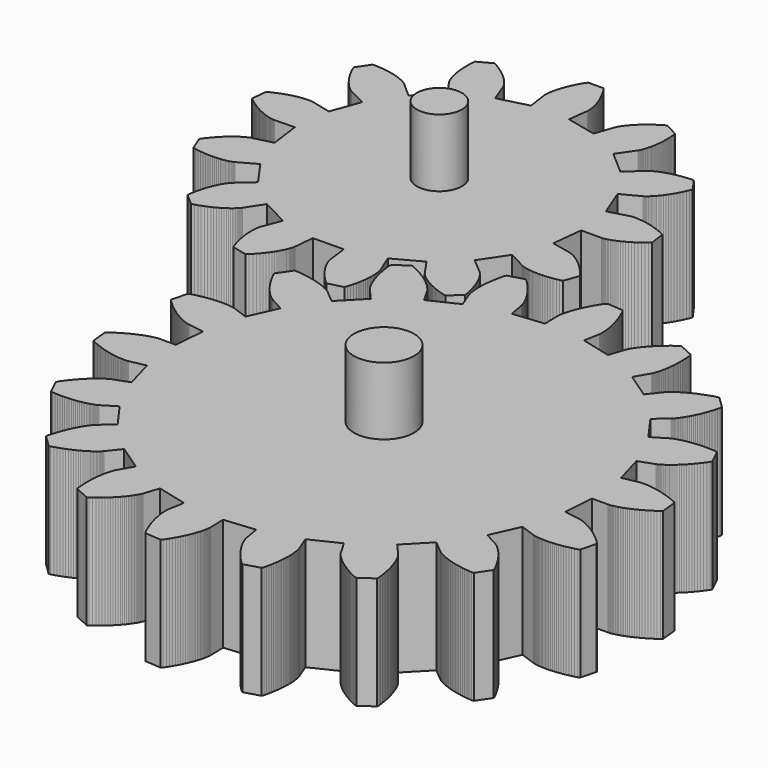
from build123d import *

# Parameters (mm, degrees)
F1_DEPTH = 25
F2_SCALE = 0.3
F3_R     = 1.5
F4_DEPTH = 12
F3_R_2   = 2


# Not quite as in the source:
# - the program builds the solid bodies; features that only make, move or delete a surface that nothing else refers to are left out


with BuildPart() as f1:
    # F0 (on Top) → F1 (new body)
    with BuildSketch(Plane.XY):
        Polygon((63.128658, -38.192269), (63.636659, -31.363161), (67.214568, -31.36309), (67.240708, -31.362349), (67.285548, -31.360198), (67.348975, -31.355999), (67.430963, -31.348944), (67.531399, -31.338361), (67.650141, -31.323509), (67.787089, -31.303718), (67.942102, -31.278212), (68.11496, -31.246286), (68.305495, -31.207304), (68.513461, -31.160525), (68.738673, -31.10528), (68.98082, -31.040863), (69.239687, -30.966603), (69.514891, -30.881866), (69.806179, -30.785946), (70.113202, -30.678172), (70.435603, -30.557981), (70.773002, -30.424666), (71.125005, -30.277628), (71.491224, -30.116233), (71.871164, -29.939914), (72.264438, -29.748074), (72.670593, -29.540111), (73.089091, -29.315462), (73.519448, -29.073598), (73.961158, -28.813953), (74.413704, -28.536), (74.876514, -28.239208), (75.349025, -27.923119), (75.830634, -27.587239), (76.133425, -27.244269), (75.778317, -23.714939), (75.413266, -23.439137), (74.874361, -23.205951), (74.348371, -22.990333), (73.835713, -22.791719), (73.336885, -22.609474), (72.852311, -22.443034), (72.382373, -22.291763), (71.927502, -22.154991), (71.48808, -22.032083), (71.064468, -21.922439), (70.65701, -21.825355), (70.265992, -21.740159), (69.891763, -21.666217), (69.534539, -21.602787), (69.194675, -21.549201), (68.872343, -21.504786), (68.567786, -21.468802), (68.281191, -21.44058), (68.012727, -21.419379), (67.762608, -21.404491), (67.530903, -21.395213), (67.317792, -21.390803), (67.123306, -21.390556), (66.947552, -21.393731), (66.790563, -21.399623), (66.652415, -21.40749), (66.533069, -21.416592), (66.432564, -21.426222), (66.350824, -21.435641), (66.287821, -21.444144), (66.243477, -21.451022), (66.217687, -21.455503), (62.7115, -22.168184), (60.853173, -15.577202), (64.215252, -14.353416), (64.239594, -14.34375), (64.28101, -14.326429), (64.339184, -14.300782), (64.413792, -14.266103), (64.504527, -14.22183), (64.611067, -14.167255), (64.732985, -14.101779), (64.869901, -14.024803), (65.021421, -13.935727), (65.187119, -13.833915), (65.366576, -13.718804), (65.559297, -13.589863), (65.764829, -13.44653), (65.982667, -13.288204), (66.212288, -13.114425), (66.453202, -12.924665), (66.704872, -12.718397), (66.966704, -12.495194), (67.238135, -12.254493), (67.518625, -11.995943), (67.80755, -11.719047), (68.104307, -11.423421), (68.408262, -11.108637), (68.71874, -10.774309), (69.035183, -10.420085), (69.356879, -10.045576), (69.68313, -9.650535), (70.013332, -9.23454), (70.346704, -8.797413), (70.682622, -8.338767), (71.020301, -7.858424), (71.187549, -7.432551), (69.646757, -4.237548), (69.209386, -4.10321), (68.623246, -4.068391), (68.055204, -4.045672), (67.505539, -4.034384), (66.974467, -4.033749), (66.462165, -4.043096), (65.968838, -4.061654), (65.494637, -4.088711), (65.03969, -4.123531), (64.604117, -4.16537), (64.188014, -4.213488), (63.791457, -4.267181), (63.414483, -4.325672), (63.057119, -4.388219), (62.719402, -4.454118), (62.401337, -4.522629), (62.102816, -4.593006), (61.823877, -4.664481), (61.564372, -4.736376), (61.324236, -4.807956), (61.103327, -4.878475), (60.901538, -4.947232), (60.718693, -5.013518), (60.554652, -5.076595), (60.409132, -5.135827), (60.282024, -5.190472), (60.172982, -5.239825), (60.081824, -5.283287), (60.008233, -5.320083), (59.95193, -5.349646), (59.912597, -5.371234), (59.889913, -5.384288), (56.83895, -7.253163), (52.838414, -1.695255), (55.579181, 0.604645), (55.598759, 0.622037), (55.631743, 0.65248), (55.677641, 0.696472), (55.735884, 0.754573), (55.806016, 0.827246), (55.887436, 0.914948), (55.979619, 1.018169), (56.08196, 1.13734), (56.193896, 1.272875), (56.314792, 1.425204), (56.444051, 1.594714), (56.581033, 1.781828), (56.725143, 1.986828), (56.875673, 2.210064), (57.032026, 2.451929), (57.193526, 2.712631), (57.359437, 2.992526), (57.529159, 3.291859), (57.701914, 3.61084), (57.877068, 3.949754), (58.053847, 4.308776), (58.231576, 4.688046), (58.409515, 5.087815), (58.586965, 5.508184), (58.763176, 5.949263), (58.937377, 6.411189), (59.108862, 6.894038), (59.276856, 7.39784), (59.440616, 7.922665), (59.5994, 8.468519), (59.752435, 9.035399), (59.763936, 9.492776), (57.223302, 11.968147), (56.766382, 11.944758), (56.203666, 11.777011), (55.662119, 11.604078), (55.141734, 11.426701), (54.642484, 11.245656), (54.164259, 11.061648), (53.707024, 10.875486), (53.270674, 10.687879), (52.855066, 10.499567), (52.460096, 10.311255), (52.085515, 10.123718), (51.731257, 9.937626), (51.396999, 9.75376), (51.082605, 9.57275), (50.787823, 9.395301), (50.512339, 9.222158), (50.255905, 9.053919), (50.018202, 8.891359), (49.798951, 8.735043), (49.597763, 8.585642), (49.414317, 8.443825), (49.248231, 8.310193), (49.099075, 8.185381), (48.9665, 8.069986), (48.850016, 7.964577), (48.749225, 7.869751), (48.663677, 7.78607), (48.592874, 7.71407), (48.536324, 7.654308), (48.493532, 7.607283), (48.463934, 7.573521), (48.447072, 7.553521), (46.219279, 4.753804), (40.559138, 8.608325), (42.348004, 11.706914), (42.360419, 11.729951), (42.381023, 11.769814), (42.409068, 11.826857), (42.443958, 11.901401), (42.485022, 11.993651), (42.531552, 12.103929), (42.582846, 12.232447), (42.638269, 12.379413), (42.697075, 12.545079), (42.758565, 12.729545), (42.822065, 12.933064), (42.8868, 13.155736), (42.952098, 13.397635), (43.017222, 13.658938), (43.081427, 13.939678), (43.143974, 14.239891), (43.204193, 14.55965), (43.261274, 14.898986), (43.314509, 15.257836), (43.36319, 15.636188), (43.406512, 16.034016), (43.4438, 16.451212), (43.474316, 16.887738), (43.497282, 17.343454), (43.511994, 17.818188), (43.517673, 18.311832), (43.513687, 18.824204), (43.499223, 19.355099), (43.473646, 19.904269), (43.436145, 20.471504), (43.386086, 21.056545), (43.240423, 21.490288), (40.006405, 22.947402), (39.585012, 22.769145), (39.11363, 22.419048), (38.663909, 22.071347), (38.235566, 21.726686), (37.82832, 21.385794), (37.441886, 21.049354), (37.075915, 20.718022), (36.730016, 20.392476), (36.403909, 20.07339), (36.097134, 19.761324), (35.809301, 19.45702), (35.540027, 19.160968), (35.288848, 18.873841), (35.05531, 18.596241), (34.838986, 18.32866), (34.63935, 18.071731), (34.455905, 17.82595), (34.28816, 17.591883), (34.135582, 17.370019), (33.997612, 17.160821), (33.873751, 16.964822), (33.763367, 16.782431), (33.665895, 16.614122), (33.580805, 16.460347), (33.507392, 16.321461), (33.445126, 16.197879), (33.393338, 16.089967), (33.351429, 15.998101), (33.318726, 15.92261), (33.294596, 15.863801), (33.278369, 15.82196), (33.269337, 15.79737), (32.133464, 12.404568), (25.496337, 14.09074), (26.117544, 17.614281), (26.121354, 17.640179), (26.127033, 17.684696), (26.133913, 17.747913), (26.141215, 17.829864), (26.148235, 17.930584), (26.154233, 18.050107), (26.158501, 18.188428), (26.160265, 18.345519), (26.158889, 18.521273), (26.153563, 18.715689), (26.143614, 18.928628), (26.128339, 19.160015), (26.106925, 19.409677), (26.078774, 19.677468), (26.043073, 19.963217), (25.999187, 20.266746), (25.946376, 20.587813), (25.88397, 20.926197), (25.811297, 21.281618), (25.727618, 21.653801), (25.632262, 22.042456), (25.524595, 22.447266), (25.40398, 22.867885), (25.269678, 23.303953), (25.121123, 23.755121), (24.957681, 24.220962), (24.778681, 24.701058), (24.583525, 25.194982), (24.371611, 25.702278), (24.142376, 26.222482), (23.895255, 26.75511), (23.610034, 27.112862), (20.072697, 27.375997), (19.737699, 27.064388), (19.414448, 26.574205), (19.110777, 26.093614), (18.826156, 25.623256), (18.560056, 25.163659), (18.311983, 24.715312), (18.081407, 24.278786), (17.86773, 23.854603), (17.670421, 23.443194), (17.488846, 23.045049), (17.322476, 22.66063), (17.170711, 22.290353), (17.032881, 21.934646), (16.908386, 21.5939), (16.79659, 21.268462), (16.69686, 20.958759), (16.60856, 20.665069), (16.530984, 20.387718), (16.463498, 20.127048), (16.405395, 19.88328), (16.356041, 19.656728), (16.314696, 19.4476), (16.280688, 19.256112), (16.253277, 19.082473), (16.231828, 18.926863), (16.215565, 18.789457), (16.203818, 18.670359), (16.195845, 18.569676), (16.190941, 18.487548), (16.188401, 18.424013), (16.187449, 18.379141), (16.187378, 18.352964), (16.280406, 14.776292), (9.466821, 14.09074), (8.845438, 17.614249), (8.840181, 17.639893), (8.830304, 17.683673), (8.815134, 17.74541), (8.793967, 17.824927), (8.766098, 17.921977), (8.730855, 18.036349), (8.68757, 18.16779), (8.635535, 18.315993), (8.574116, 18.480707), (8.502608, 18.661574), (8.420446, 18.858246), (8.326925, 19.070442), (8.221444, 19.297738), (8.10337, 19.539745), (7.972101, 19.796071), (7.827039, 20.066301), (7.667619, 20.349935), (7.493241, 20.646547), (7.303375, 20.95569), (7.097424, 21.276789), (6.874927, 21.609419), (6.63532, 21.952992), (6.378075, 22.30697), (6.102766, 22.670826), (5.808867, 23.043956), (5.495918, 23.425802), (5.163496, 23.815695), (4.811212, 24.213098), (4.438573, 24.617348), (4.045226, 25.027766), (3.630818, 25.443761), (3.240469, 25.682383), (-0.173573, 24.719828), (-0.381782, 24.312403), (-0.517849, 23.741222), (-0.638852, 23.185776), (-0.74546, 22.646414), (-0.838277, 22.123524), (-0.918039, 21.617396), (-0.985456, 21.128338), (-1.04116, 20.65664), (-1.085856, 20.202544), (-1.120287, 19.766336), (-1.145122, 19.348187), (-1.161139, 18.948314), (-1.169007, 18.566926), (-1.169429, 18.20413), (-1.163185, 17.860132), (-1.150944, 17.53498), (-1.133482, 17.228802), (-1.111538, 16.941643), (-1.085786, 16.673603), (-1.056999, 16.424679), (-1.025919, 16.19488), (-0.993252, 15.98424), (-0.959704, 15.792644), (-0.926048, 15.620136), (-0.892993, 15.466571), (-0.861277, 15.331884), (-0.831574, 15.215924), (-0.804657, 15.118627), (-0.781162, 15.039745), (-0.76183, 14.979176), (-0.747401, 14.936699), (-0.738511, 14.912078), (0.5722, 11.582912), (-5.59598, 8.608325), (-7.384986, 11.706807), (-7.39871, 11.729103), (-7.422944, 11.766886), (-7.458329, 11.819695), (-7.505424, 11.887184), (-7.564795, 11.968852), (-7.637046, 12.064278), (-7.722664, 12.172968), (-7.822254, 12.294464), (-7.936306, 12.428204), (-8.065352, 12.573724), (-8.209852, 12.730463), (-8.370294, 12.897857), (-8.547178, 13.075373), (-8.740886, 13.26238), (-8.95192, 13.45835), (-9.180626, 13.662679), (-9.427464, 13.874662), (-9.692753, 14.093771), (-9.976914, 14.319306), (-10.280233, 14.550623), (-10.603095, 14.787085), (-10.945783, 15.028), (-11.308581, 15.27265), (-11.691732, 15.520406), (-12.095521, 15.770488), (-12.520197, 16.02227), (-12.965895, 16.274995), (-13.432902, 16.527903), (-13.921287, 16.780315), (-14.431299, 17.031495), (-14.962971, 17.280662), (-15.41142, 17.371359), (-18.290336, 15.299177), (-18.346639, 14.845157), (-18.279188, 14.261837), (-18.202917, 13.698521), (-18.118603, 13.155243), (-18.026985, 12.632108), (-17.928843, 12.129224), (-17.824879, 11.646625), (-17.715907, 11.184309), (-17.602595, 10.742314), (-17.485755, 10.320637), (-17.366127, 9.919211), (-17.244383, 9.537966), (-17.121299, 9.176898), (-16.99765, 8.835831), (-16.874108, 8.514697), (-16.751412, 8.213356), (-16.630303, 7.931593), (-16.511453, 7.669303), (-16.395566, 7.426203), (-16.283382, 7.202153), (-16.175572, 6.996871), (-16.072844, 6.810077), (-15.975794, 6.641518), (-15.885167, 6.490919), (-15.801593, 6.357922), (-15.72571, 6.24221), (-15.658154, 6.143397), (-15.599557, 6.061164), (-15.550521, 5.995089), (-15.511646, 5.944782), (-15.483528, 5.909787), (-15.466736, 5.889714), (-13.096459, 3.209627), (-17.875256, -1.695255), (-20.616163, 0.604502), (-20.636658, 0.620766), (-20.672361, 0.647964), (-20.72369, 0.685502), (-20.790999, 0.732807), (-20.87475, 0.789253), (-20.975255, 0.854199), (-21.092908, 0.927049), (-21.22802, 1.007164), (-21.38095, 1.09384), (-21.551977, 1.186446), (-21.741382, 1.284305), (-21.94938, 1.386716), (-22.176288, 1.493043), (-22.422316, 1.602546), (-22.68764, 1.714517), (-22.972436, 1.828254), (-23.276883, 1.943083), (-23.601123, 2.05823), (-23.945291, 2.172954), (-24.309464, 2.286583), (-24.693711, 2.398342), (-25.0981, 2.507527), (-25.522703, 2.613361), (-25.967484, 2.715102), (-26.43248, 2.812046), (-26.917622, 2.903379), (-27.422904, 2.988398), (-27.948228, 3.066362), (-28.493516, 3.136494), (-29.058663, 3.198091), (-29.6435, 3.250373), (-30.095938, 3.182252), (-32.092484, 0.250384), (-31.990105, -0.195527), (-31.727218, -0.720565), (-31.462844, -1.223837), (-31.197841, -1.705521), (-30.932832, -2.165756), (-30.668599, -2.604753), (-30.405851, -3.022723), (-30.145327, -3.419881), (-29.887693, -3.79647), (-29.633655, -4.152742), (-29.383928, -4.489045), (-29.13917, -4.805628), (-28.900021, -5.102842), (-28.667155, -5.381042), (-28.441232, -5.640547), (-28.222861, -5.881776), (-28.012678, -6.105118), (-27.811312, -6.310965), (-27.619296, -6.499737), (-27.437229, -6.671927), (-27.265706, -6.827961), (-27.105264, -6.968329), (-26.956463, -7.093532), (-26.81976, -7.204057), (-26.695758, -7.300472), (-26.584845, -7.383232), (-26.487585, -7.452976), (-26.4044, -7.510197), (-26.335713, -7.55553), (-26.281986, -7.589502), (-26.243603, -7.612786), (-26.220956, -7.625909), (-23.076965, -9.33367), (-25.890015, -15.577202), (-29.252164, -14.353556), (-29.277001, -14.345302), (-29.31986, -14.331967), (-29.380924, -14.314222), (-29.460372, -14.292808), (-29.558342, -14.268432), (-29.675001, -14.241762), (-29.810469, -14.21354), (-29.964847, -14.184471), (-30.1382, -14.155331), (-30.33057, -14.126791), (-30.542024, -14.099627), (-30.772528, -14.07451), (-31.02212, -14.052214), (-31.290762, -14.033481), (-31.578379, -14.018982), (-31.884906, -14.009492), (-32.210241, -14.005754), (-32.554342, -14.008469), (-32.91696, -14.018347), (-33.29803, -14.036127), (-33.697338, -14.062516), (-34.114712, -14.098252), (-34.549865, -14.144007), (-35.002653, -14.200521), (-35.472731, -14.268467), (-35.959878, -14.348582), (-36.46375, -14.44147), (-36.984062, -14.547903), (-37.520463, -14.668481), (-38.072561, -14.803912), (-38.640038, -14.954795), (-39.041887, -15.173554), (-39.915262, -18.611479), (-39.666553, -18.995478), (-39.239937, -19.39895), (-38.819393, -19.781466), (-38.405616, -20.143452), (-37.999181, -20.485293), (-37.600755, -20.80745), (-37.2109, -21.11031), (-36.830254, -21.394402), (-36.459341, -21.660185), (-36.098769, -21.908116), (-35.749097, -22.138692), (-35.410784, -22.352475), (-35.084425, -22.549996), (-34.770453, -22.731747), (-34.469395, -22.898364), (-34.181703, -23.050341), (-33.907807, -23.188312), (-33.64816, -23.312843), (-33.40316, -23.424602), (-33.173183, -23.524121), (-32.958656, -23.612104), (-32.759869, -23.689115), (-32.577198, -23.755861), (-32.410972, -23.813011), (-32.261466, -23.861165), (-32.128926, -23.901029), (-32.013672, -23.933273), (-31.915917, -23.958602), (-31.83591, -23.977688), (-31.773786, -23.99127), (-31.729758, -23.999983), (-31.704006, -24.004604), (-28.1655, -24.534053), (-28.673501, -31.363161), (-32.25141, -31.363231), (-32.27755, -31.363972), (-32.32239, -31.366124), (-32.385818, -31.370322), (-32.467805, -31.377378), (-32.568241, -31.387961), (-32.686983, -31.402813), (-32.823931, -31.422604), (-32.978945, -31.44811), (-33.151802, -31.480036), (-33.342338, -31.519018), (-33.550303, -31.565796), (-33.775515, -31.621041), (-34.017662, -31.685459), (-34.276529, -31.759718), (-34.551733, -31.844456), (-34.843021, -31.940376), (-35.150044, -32.048149), (-35.472445, -32.168341), (-35.809844, -32.301656), (-36.161847, -32.448693), (-36.528066, -32.610089), (-36.908006, -32.786408), (-37.30128, -32.978248), (-37.707435, -33.186211), (-38.125933, -33.41086), (-38.55629, -33.652724), (-38.998, -33.912368), (-39.450546, -34.190322), (-39.913357, -34.487114), (-40.385868, -34.803203), (-40.867476, -35.139082), (-41.170267, -35.482053), (-40.815159, -39.011383), (-40.450108, -39.287185), (-39.911203, -39.520371), (-39.385213, -39.735988), (-38.872556, -39.934603), (-38.373727, -40.116848), (-37.889153, -40.283288), (-37.419215, -40.434559), (-36.964344, -40.571331), (-36.524922, -40.694239), (-36.10131, -40.803883), (-35.693852, -40.900967), (-35.302834, -40.986162), (-34.928605, -41.060105), (-34.571381, -41.123534), (-34.231517, -41.177121), (-33.909185, -41.221536), (-33.604628, -41.25752), (-33.318033, -41.285742), (-33.049569, -41.306943), (-32.79945, -41.32183), (-32.567745, -41.331109), (-32.354634, -41.335519), (-32.160148, -41.335766), (-31.984394, -41.33259), (-31.827405, -41.326699), (-31.689257, -41.318832), (-31.569911, -41.30973), (-31.469406, -41.300099), (-31.387666, -41.290681), (-31.324664, -41.282178), (-31.280319, -41.275299), (-31.254529, -41.270819), (-27.748342, -40.558138), (-25.890015, -47.14912), (-29.252094, -48.372905), (-29.276436, -48.382572), (-29.317852, -48.399893), (-29.376026, -48.42554), (-29.450634, -48.460218), (-29.541369, -48.504492), (-29.647909, -48.559067), (-29.769827, -48.624543), (-29.906743, -48.701519), (-30.058263, -48.790595), (-30.223961, -48.892407), (-30.403418, -49.007517), (-30.596139, -49.136458), (-30.801671, -49.279792), (-31.019509, -49.438118), (-31.24913, -49.611896), (-31.490044, -49.801656), (-31.741714, -50.007925), (-32.003546, -50.231128), (-32.274977, -50.471828), (-32.555467, -50.730379), (-32.844392, -51.007274), (-33.141149, -51.302901), (-33.445104, -51.617685), (-33.755582, -51.952012), (-34.072025, -52.306237), (-34.393721, -52.680746), (-34.719972, -53.075786), (-35.050174, -53.491782), (-35.383546, -53.928909), (-35.719464, -54.387555), (-36.057143, -54.867898), (-36.224391, -55.293771), (-34.683599, -58.488774), (-34.246228, -58.623111), (-33.660088, -58.657931), (-33.092046, -58.68065), (-32.542381, -58.691938), (-32.011309, -58.692573), (-31.499007, -58.683226), (-31.00568, -58.664668), (-30.531479, -58.63761), (-30.076532, -58.602791), (-29.640959, -58.560952), (-29.224856, -58.512833), (-28.828299, -58.459141), (-28.451325, -58.40065), (-28.093961, -58.338102), (-27.756244, -58.272204), (-27.438179, -58.203693), (-27.139658, -58.133316), (-26.860719, -58.061841), (-26.601214, -57.989946), (-26.361078, -57.918366), (-26.140169, -57.847846), (-25.938381, -57.77909), (-25.755535, -57.712804), (-25.591494, -57.649727), (-25.445974, -57.590495), (-25.318866, -57.53585), (-25.209824, -57.486496), (-25.118666, -57.443034), (-25.045075, -57.406239), (-24.988772, -57.376676), (-24.949439, -57.355087), (-24.926755, -57.342034), (-21.875792, -55.473158), (-17.875256, -61.031066), (-20.616023, -63.330966), (-20.635601, -63.348359), (-20.668585, -63.378802), (-20.714483, -63.422794), (-20.772726, -63.480895), (-20.842858, -63.553568), (-20.924278, -63.64127), (-21.016461, -63.744491), (-21.118802, -63.863661), (-21.230738, -63.999196), (-21.351634, -64.151526), (-21.480893, -64.321036), (-21.617876, -64.50815), (-21.761985, -64.713149), (-21.912515, -64.936386), (-22.068868, -65.178251), (-22.230368, -65.438953), (-22.396279, -65.718848), (-22.566001, -66.018181), (-22.738756, -66.337162), (-22.91391, -66.676076), (-23.090689, -67.035098), (-23.268418, -67.414368), (-23.446357, -67.814136), (-23.623807, -68.234505), (-23.800018, -68.675585), (-23.974219, -69.137511), (-24.145704, -69.620359), (-24.313698, -70.124162), (-24.477458, -70.648987), (-24.636242, -71.194841), (-24.789277, -71.76172), (-24.800778, -72.219097), (-22.260144, -74.694468), (-21.803224, -74.671079), (-21.240508, -74.503333), (-20.698961, -74.3304), (-20.178577, -74.153023), (-19.679326, -73.971978), (-19.201101, -73.78797), (-18.743867, -73.601808), (-18.307516, -73.414201), (-17.891908, -73.225889), (-17.496938, -73.037577), (-17.122357, -72.85004), (-16.768099, -72.663948), (-16.433841, -72.480082), (-16.119447, -72.299072), (-15.824665, -72.121623), (-15.549181, -71.94848), (-15.292747, -71.780241), (-15.055044, -71.617681), (-14.835793, -71.461365), (-14.634605, -71.311963), (-14.451159, -71.170146), (-14.285073, -71.036514), (-14.135917, -70.911702), (-14.003342, -70.796308), (-13.886858, -70.690899), (-13.786067, -70.596072), (-13.700519, -70.512392), (-13.629716, -70.440392), (-13.573166, -70.38063), (-13.530374, -70.333605), (-13.500776, -70.299843), (-13.483914, -70.279842), (-11.256121, -67.480126), (-5.59598, -71.334647), (-7.384846, -74.433236), (-7.397262, -74.456272), (-7.417865, -74.496136), (-7.44591, -74.553179), (-7.4808, -74.627722), (-7.521864, -74.719973), (-7.568394, -74.830251), (-7.619688, -74.958769), (-7.675111, -75.105735), (-7.733917, -75.271401), (-7.795407, -75.455867), (-7.858907, -75.659386), (-7.923642, -75.882057), (-7.988941, -76.123957), (-8.054064, -76.385259), (-8.118269, -76.666), (-8.180816, -76.966213), (-8.241035, -77.285971), (-8.298116, -77.625308), (-8.351351, -77.984158), (-8.400032, -78.36251), (-8.443354, -78.760338), (-8.480642, -79.177533), (-8.511158, -79.614059), (-8.534124, -80.069775), (-8.548836, -80.54451), (-8.554515, -81.038154), (-8.550529, -81.550526), (-8.536065, -82.081421), (-8.510488, -82.63059), (-8.472987, -83.197825), (-8.422928, -83.782867), (-8.277265, -84.21661), (-5.043247, -85.673724), (-4.621854, -85.495467), (-4.150472, -85.14537), (-3.700751, -84.797668), (-3.272408, -84.453008), (-2.865162, -84.112116), (-2.478728, -83.775675), (-2.112757, -83.444343), (-1.766859, -83.118798), (-1.440751, -82.799712), (-1.133976, -82.487646), (-0.846143, -82.183342), (-0.576869, -81.887289), (-0.32569, -81.600162), (-0.092152, -81.322563), (0.124172, -81.054981), (0.323808, -80.798053), (0.507253, -80.552272), (0.674998, -80.318205), (0.827576, -80.09634), (0.965546, -79.887142), (1.089407, -79.691143), (1.199791, -79.508752), (1.297263, -79.340443), (1.382353, -79.186668), (1.455766, -79.047783), (1.518032, -78.9242), (1.56982, -78.816288), (1.611729, -78.724423), (1.644432, -78.648932), (1.668562, -78.590123), (1.684789, -78.548281), (1.693821, -78.523692), (2.829694, -75.130889), (9.466821, -76.817062), (8.845614, -80.340603), (8.841804, -80.3665), (8.836125, -80.411018), (8.829245, -80.474235), (8.821943, -80.556185), (8.814923, -80.656906), (8.808925, -80.776429), (8.804657, -80.91475), (8.802893, -81.071841), (8.804269, -81.247594), (8.809595, -81.442011), (8.819544, -81.65495), (8.834819, -81.886337), (8.856233, -82.135998), (8.884384, -82.40379), (8.920085, -82.689539), (8.963971, -82.993068), (9.016782, -83.314135), (9.079188, -83.652519), (9.151861, -84.007939), (9.23554, -84.380123), (9.330896, -84.768778), (9.438563, -85.173588), (9.559178, -85.594207), (9.69348, -86.030275), (9.842035, -86.481443), (10.005477, -86.947284), (10.184476, -87.42738), (10.379633, -87.921304), (10.591547, -88.4286), (10.820782, -88.948804), (11.067903, -89.481432), (11.353124, -89.839183), (14.890461, -90.102319), (15.225459, -89.79071), (15.54871, -89.300527), (15.852381, -88.819936), (16.137002, -88.349578), (16.403102, -87.889981), (16.651175, -87.441634), (16.881751, -87.005108), (17.095428, -86.580925), (17.292737, -86.169516), (17.474312, -85.771371), (17.640682, -85.386952), (17.792447, -85.016674), (17.930277, -84.660968), (18.054772, -84.320221), (18.166568, -83.994784), (18.266298, -83.68508), (18.354598, -83.391391), (18.432174, -83.114039), (18.49966, -82.85337), (18.557763, -82.609602), (18.607116, -82.383049), (18.648462, -82.173921), (18.68247, -81.982433), (18.709881, -81.808795), (18.73133, -81.653184), (18.747593, -81.515779), (18.75934, -81.396681), (18.767313, -81.295998), (18.772216, -81.21387), (18.774756, -81.150335), (18.775709, -81.105463), (18.77578, -81.079285), (18.682752, -77.502614), (25.496337, -76.817062), (26.11772, -80.340571), (26.122977, -80.366215), (26.132854, -80.409995), (26.148024, -80.471732), (26.169191, -80.551249), (26.19706, -80.648299), (26.232303, -80.76267), (26.275588, -80.894111), (26.327623, -81.042315), (26.389042, -81.207028), (26.46055, -81.387896), (26.542712, -81.584568), (26.636233, -81.796764), (26.741714, -82.02406), (26.859788, -82.266067), (26.991057, -82.522393), (27.136119, -82.792623), (27.295539, -83.076256), (27.469917, -83.372868), (27.659783, -83.682012), (27.865734, -84.003111), (28.088231, -84.33574), (28.327838, -84.679313), (28.585083, -85.033291), (28.860392, -85.397147), (29.154291, -85.770278), (29.46724, -86.152124), (29.799662, -86.542017), (30.151946, -86.93942), (30.524585, -87.343669), (30.917932, -87.754088), (31.33234, -88.170083), (31.722689, -88.408704), (35.136731, -87.44615), (35.34494, -87.038725), (35.481007, -86.467544), (35.60201, -85.912098), (35.708618, -85.372736), (35.801435, -84.849845), (35.881197, -84.343718), (35.948614, -83.85466), (36.004318, -83.382961), (36.049014, -82.928866), (36.083445, -82.492657), (36.10828, -82.074509), (36.124297, -81.674636), (36.132165, -81.293247), (36.132587, -80.930452), (36.126343, -80.586454), (36.114102, -80.261301), (36.09664, -79.955124), (36.074696, -79.667964), (36.048944, -79.399925), (36.020157, -79.151001), (35.989077, -78.921202), (35.95641, -78.710562), (35.922862, -78.518966), (35.889206, -78.346458), (35.856151, -78.192893), (35.824435, -78.058206), (35.794732, -77.942246), (35.767815, -77.844949), (35.744319, -77.766067), (35.724988, -77.705498), (35.710559, -77.663021), (35.701669, -77.638399), (34.390958, -74.309234), (40.559138, -71.334647), (42.348144, -74.433128), (42.361867, -74.455424), (42.386102, -74.493208), (42.421486, -74.546017), (42.468582, -74.613506), (42.527953, -74.695174), (42.600203, -74.7906), (42.685822, -74.89929), (42.785412, -75.020786), (42.899464, -75.154526), (43.02851, -75.300046), (43.17301, -75.456785), (43.333452, -75.624179), (43.510336, -75.801695), (43.704044, -75.988702), (43.915078, -76.184671), (44.143784, -76.389), (44.390622, -76.600984), (44.655911, -76.820092), (44.940072, -77.045628), (45.243391, -77.276944), (45.566253, -77.513407), (45.90894, -77.754321), (46.271739, -77.998972), (46.65489, -78.246728), (47.058679, -78.496809), (47.483355, -78.748592), (47.929053, -79.001317), (48.39606, -79.254224), (48.884445, -79.506637), (49.394457, -79.757817), (49.926129, -80.006983), (50.374578, -80.097681), (53.253494, -78.025499), (53.309797, -77.571478), (53.242346, -76.988159), (53.166074, -76.424843), (53.081761, -75.881565), (52.990143, -75.35843), (52.892001, -74.855545), (52.788037, -74.372947), (52.679064, -73.910631), (52.565753, -73.468636), (52.448913, -73.046959), (52.329285, -72.645533), (52.207541, -72.264287), (52.084457, -71.90322), (51.960808, -71.562153), (51.837266, -71.241019), (51.71457, -70.939678), (51.593461, -70.657915), (51.474611, -70.395624), (51.358724, -70.152524), (51.24654, -69.928475), (51.13873, -69.723193), (51.036002, -69.536399), (50.938952, -69.367839), (50.848325, -69.21724), (50.764751, -69.084243), (50.688868, -68.968531), (50.621312, -68.869719), (50.562715, -68.787486), (50.513679, -68.72141), (50.474804, -68.671104), (50.446686, -68.636109), (50.429894, -68.616036), (48.059617, -65.935948), (52.838414, -61.031066), (55.579321, -63.330824), (55.599816, -63.347088), (55.635519, -63.374286), (55.686848, -63.411824), (55.754157, -63.459129), (55.837908, -63.515575), (55.938413, -63.58052), (56.056066, -63.653371), (56.191178, -63.733485), (56.344108, -63.820162), (56.515135, -63.912768), (56.70454, -64.010627), (56.912538, -64.113038), (57.139446, -64.219365), (57.385474, -64.328868), (57.650798, -64.440839), (57.935594, -64.554575), (58.240041, -64.669405), (58.564281, -64.784552), (58.908448, -64.899276), (59.272622, -65.012905), (59.656869, -65.124663), (60.061258, -65.233849), (60.485861, -65.339683), (60.930641, -65.441424), (61.395638, -65.538368), (61.88078, -65.629701), (62.386062, -65.714719), (62.911386, -65.792683), (63.456674, -65.862815), (64.021821, -65.924413), (64.606658, -65.976695), (65.059096, -65.908573), (67.055642, -62.976705), (66.953263, -62.530794), (66.690375, -62.005756), (66.426002, -61.502485), (66.160999, -61.020801), (65.89599, -60.560566), (65.631757, -60.121569), (65.369009, -59.703598), (65.108485, -59.306441), (64.850851, -58.929851), (64.596812, -58.57358), (64.347086, -58.237277), (64.102328, -57.920694), (63.863179, -57.623479), (63.630312, -57.34528), (63.40439, -57.085775), (63.186019, -56.844546), (62.975836, -56.621204), (62.77447, -56.415357), (62.582454, -56.226585), (62.400386, -56.054394), (62.228864, -55.898361), (62.068422, -55.757992), (61.919621, -55.63279), (61.782918, -55.522264), (61.658916, -55.42585), (61.548003, -55.34309), (61.450743, -55.273345), (61.367558, -55.216125), (61.298871, -55.170792), (61.245144, -55.13682), (61.20676, -55.113536), (61.184114, -55.100412), (58.040123, -53.392652), (60.853173, -47.14912), (64.215322, -48.372765), (64.240159, -48.38102), (64.283018, -48.394355), (64.344082, -48.4121), (64.42353, -48.433513), (64.521499, -48.45789), (64.638159, -48.48456), (64.773627, -48.512782), (64.928005, -48.541851), (65.101357, -48.57099), (65.293728, -48.599531), (65.505182, -48.626694), (65.735686, -48.651811), (65.985277, -48.674108), (66.25392, -48.69284), (66.541537, -48.707339), (66.848064, -48.716829), (67.173399, -48.720568), (67.5175, -48.717852), (67.880118, -48.707975), (68.261188, -48.690195), (68.660496, -48.663806), (69.07787, -48.62807), (69.513023, -48.582315), (69.965811, -48.5258), (70.435889, -48.457855), (70.923036, -48.377739), (71.426908, -48.284852), (71.94722, -48.178419), (72.483621, -48.057841), (73.035719, -47.922409), (73.603196, -47.771526), (74.005045, -47.552768), (74.87842, -44.114843), (74.629711, -43.730844), (74.203095, -43.327372), (73.782551, -42.944856), (73.368774, -42.58287), (72.962339, -42.241028), (72.563913, -41.918872), (72.174058, -41.616012), (71.793412, -41.33192), (71.422499, -41.066137), (71.061927, -40.818205), (70.712255, -40.587629), (70.373942, -40.373846), (70.047583, -40.176326), (69.733611, -39.994574), (69.432553, -39.827958), (69.144861, -39.675981), (68.870965, -39.53801), (68.611318, -39.413479), (68.366318, -39.301719), (68.136341, -39.2022), (67.921814, -39.114218), (67.723027, -39.037207), (67.540356, -38.970461), (67.37413, -38.913311), (67.224624, -38.865156), (67.092084, -38.825293), (66.97683, -38.793049), (66.879075, -38.767719), (66.799068, -38.748634), (66.736943, -38.735052), (66.692916, -38.726339), (66.667164, -38.721717), align=None)
    extrude(amount=F1_DEPTH)


with BuildPart() as f1b:
    # F0 (on Top) → F1, piece 2 (new body)
    with BuildSketch(Plane.XY):
        Polygon((-1.427367, 39.241536), (-0.688227, 46.020408), (3.773987, 46.020478), (3.803763, 46.021466), (3.859326, 46.024712), (3.940606, 46.031661), (4.047391, 46.043656), (4.179435, 46.062106), (4.336493, 46.088353), (4.518209, 46.123736), (4.724196, 46.169597), (4.953959, 46.227277), (5.207042, 46.298079), (5.482878, 46.383275), (5.780871, 46.484134), (6.100309, 46.601927), (6.440529, 46.737852), (6.800751, 46.893109), (7.180199, 47.068863), (7.577954, 47.266278), (7.993174, 47.486376), (8.424834, 47.730286), (8.872015, 47.999068), (9.333626, 48.293637), (9.80864, 48.615018), (10.29586, 48.964127), (10.794196, 49.341846), (11.302441, 49.748951), (11.756325, 50.180328), (11.305017, 53.552108), (10.753662, 53.848934), (10.156266, 54.108085), (9.576123, 54.341448), (9.01422, 54.550116), (8.471437, 54.735254), (7.948584, 54.898096), (7.446475, 55.039771), (6.965849, 55.161586), (6.50738, 55.264773), (6.071699, 55.350604), (5.65941, 55.420383), (5.271035, 55.475452), (4.907039, 55.517115), (4.567845, 55.546748), (4.253835, 55.565693), (3.9653, 55.575359), (3.702515, 55.577122), (3.465624, 55.572325), (3.254841, 55.562412), (3.070232, 55.548759), (2.911798, 55.532778), (2.779542, 55.515845), (2.673357, 55.499335), (2.593135, 55.48466), (2.538665, 55.473194), (2.509702, 55.466315), (-1.795491, 54.29287), (-4.291323, 60.638743), (-0.340248, 62.712512), (-0.314353, 62.727222), (-0.266658, 62.755939), (-0.197936, 62.79986), (-0.108966, 62.860114), (-0.000594, 62.937795), (0.126266, 63.033998), (0.270729, 63.149779), (0.431806, 63.286128), (0.608442, 63.443997), (0.799648, 63.624301), (1.004295, 63.827925), (1.221252, 64.055713), (1.449393, 64.308478), (1.687449, 64.586926), (1.934287, 64.891832), (2.18857, 65.22376), (2.449025, 65.583382), (2.714384, 65.971261), (2.983271, 66.387857), (3.254311, 66.833626), (3.526161, 67.308994), (3.797411, 67.814313), (4.066581, 68.349865), (4.33233, 68.915896), (4.593137, 69.512552), (4.794538, 70.105463), (2.82798, 72.881295), (2.201834, 72.887892), (1.552442, 72.839704), (0.930352, 72.776734), (0.335817, 72.700393), (-0.23085, 72.61209), (-0.769472, 72.513278), (-1.279906, 72.405398), (-1.76212, 72.289899), (-2.216003, 72.16819), (-2.641663, 72.04172), (-3.039174, 71.911899), (-3.408639, 71.78017), (-3.750303, 71.647913), (-4.064418, 71.516539), (-4.35126, 71.387389), (-4.611257, 71.261869), (-4.844762, 71.14129), (-5.052264, 71.026954), (-5.2343, 70.920239), (-5.391426, 70.822345), (-5.524282, 70.734538), (-5.633503, 70.658092), (-5.719862, 70.594131), (-5.784102, 70.54386), (-5.827001, 70.508408), (-5.849438, 70.488827), (-9.11616, 67.449082), (-14.275217, 71.908193), (-11.740403, 75.580576), (-11.724316, 75.605623), (-11.695424, 75.653246), (-11.654995, 75.724051), (-11.60423, 75.818769), (-11.544365, 75.937902), (-11.476737, 76.082085), (-11.402618, 76.251734), (-11.323385, 76.447278), (-11.240305, 76.669178), (-11.154792, 76.917674), (-11.06822, 77.193088), (-10.981966, 77.495594), (-10.89744, 77.82544), (-10.816054, 78.18263), (-10.739184, 78.567299), (-10.668311, 78.979413), (-10.604775, 79.418867), (-10.550095, 79.885629), (-10.505611, 80.379446), (-10.472766, 80.900145), (-10.452976, 81.447409), (-10.447648, 82.020886), (-10.458161, 82.620184), (-10.48589, 83.244847), (-10.532244, 83.894383), (-10.629435, 84.512979), (-13.660749, 86.056947), (-14.218243, 85.771795), (-14.77087, 85.42738), (-15.292451, 85.082504), (-15.783377, 84.738617), (-16.244105, 84.397092), (-16.675129, 84.059271), (-17.076943, 83.726531), (-17.450217, 83.400176), (-17.795586, 83.081477), (-18.113722, 82.771669), (-18.405363, 82.472018), (-18.671286, 82.183658), (-18.912374, 81.907749), (-19.12944, 81.645459), (-19.323396, 81.397811), (-19.49527, 81.165824), (-19.645976, 80.950559), (-19.77661, 80.752897), (-19.888194, 80.573792), (-19.981821, 80.414088), (-20.058656, 80.274637), (-20.119863, 80.156139), (-20.166606, 80.059407), (-20.20012, 79.985042), (-20.221603, 79.933677), (-20.232399, 79.905947), (-21.712302, 75.69625), (-28.352638, 77.247063), (-27.814863, 81.676785), (-27.812253, 81.706456), (-27.808795, 81.762016), (-27.805903, 81.843509), (-27.80495, 81.950966), (-27.807314, 82.084281), (-27.81444, 82.243347), (-27.827634, 82.428026), (-27.848342, 82.638034), (-27.877905, 82.873092), (-27.917698, 83.132841), (-27.969027, 83.416933), (-28.033233, 83.724908), (-28.111691, 84.056237), (-28.2056, 84.410356), (-28.316302, 84.786665), (-28.44503, 85.184528), (-28.593056, 85.603169), (-28.761507, 86.041883), (-28.951619, 86.499822), (-29.164521, 86.976109), (-29.401305, 87.469891), (-29.663101, 87.98015), (-29.950933, 88.505928), (-30.265787, 89.046173), (-30.608687, 89.599751), (-30.982208, 90.102318), (-34.383832, 90.060727), (-34.744936, 89.549165), (-35.074219, 88.987364), (-35.375773, 88.439607), (-35.650657, 87.906947), (-35.899895, 87.390447), (-36.124544, 86.891018), (-36.325733, 86.409652), (-36.504591, 85.947197), (-36.662283, 85.504496), (-36.800007, 85.082362), (-36.918964, 84.681501), (-37.020423, 84.302583), (-37.105689, 83.946242), (-37.175998, 83.613112), (-37.232654, 83.303691), (-37.277033, 83.0184), (-37.310442, 82.757733), (-37.334254, 82.522042), (-37.349812, 82.311574), (-37.358525, 82.126648), (-37.361735, 81.967476), (-37.360854, 81.834127), (-37.357255, 81.726739), (-37.352387, 81.645319), (-37.347589, 81.589861), (-37.344238, 81.560263), (-36.698266, 77.145039), (-43.298703, 75.432302), (-44.881123, 79.604533), (-44.892589, 79.632016), (-44.915343, 79.682815), (-44.950656, 79.756336), (-44.999727, 79.851937), (-45.063826, 79.968847), (-45.144049, 80.106433), (-45.241557, 80.263771), (-45.357479, 80.440088), (-45.492875, 80.634504), (-45.648839, 80.84603), (-45.82632, 81.073713), (-46.026311, 81.316566), (-46.249725, 81.573494), (-46.497445, 81.843404), (-46.770354, 82.125167), (-47.069227, 82.417621), (-47.394841, 82.719527), (-47.747902, 83.02969), (-48.129042, 83.346836), (-48.5389, 83.669663), (-48.978037, 83.996828), (-49.446985, 84.32696), (-49.946166, 84.658747), (-50.476038, 84.990781), (-51.036919, 85.321616), (-51.601222, 85.593008), (-54.593871, 83.97538), (-54.675893, 83.354598), (-54.706338, 82.704145), (-54.71879, 82.078989), (-54.714662, 81.479583), (-54.695331, 80.906427), (-54.662169, 80.359795), (-54.61659, 79.840084), (-54.56004, 79.347465), (-54.49393, 78.882223), (-54.419706, 78.444425), (-54.338743, 78.034181), (-54.252524, 77.651522), (-54.162389, 77.296381), (-54.06982, 76.968756), (-53.976193, 76.6684), (-53.882918, 76.395209), (-53.791373, 76.148866), (-53.702896, 75.929085), (-53.6189, 75.735514), (-53.540653, 75.567735), (-53.469534, 75.425248), (-53.406775, 75.307595), (-53.353717, 75.214179), (-53.31156, 75.144365), (-53.281503, 75.097482), (-53.264817, 75.072858), (-50.640961, 71.463517), (-55.689424, 66.879593), (-59.029487, 69.838587), (-59.052419, 69.857567), (-59.096198, 69.891962), (-59.161639, 69.94068), (-59.249516, 70.002487), (-59.360604, 70.076253), (-59.495541, 70.160779), (-59.655033, 70.254795), (-59.839607, 70.357031), (-60.049862, 70.466251), (-60.286223, 70.581077), (-60.549218, 70.700213), (-60.839131, 70.82231), (-61.156349, 70.945956), (-61.501155, 71.069853), (-61.873758, 71.192512), (-62.274301, 71.312563), (-62.702928, 71.428558), (-63.159669, 71.539153), (-63.644526, 71.642834), (-64.157466, 71.738191), (-64.698343, 71.82381), (-65.266986, 71.89821), (-65.863216, 71.960017), (-66.486682, 72.007748), (-67.137062, 72.040027), (-67.762855, 72.018118), (-69.660939, 69.195016), (-69.445074, 68.607215), (-69.169768, 68.017126), (-68.890298, 67.457761), (-68.608074, 66.928947), (-68.324546, 66.430437), (-68.04116, 65.961842), (-67.759292, 65.522809), (-67.480314, 65.112917), (-67.205571, 64.73167), (-66.936366, 64.37854), (-66.674041, 64.052891), (-66.419866, 63.754123), (-66.175038, 63.481567), (-65.940793, 63.234481), (-65.718331, 63.012055), (-65.50878, 62.813477), (-65.313201, 62.637898), (-65.132754, 62.484406), (-64.968396, 62.352078), (-64.821147, 62.239859), (-64.691959, 62.146762), (-64.581716, 62.071727), (-64.491298, 62.013694), (-64.421519, 61.971466), (-64.373153, 61.943915), (-64.346906, 61.929838), (-60.346302, 59.953331), (-62.686206, 53.548333), (-67.018812, 54.616156), (-67.04795, 54.622329), (-67.102667, 54.632454), (-67.18324, 54.645154), (-67.289779, 54.659053), (-67.422423, 54.672741), (-67.58121, 54.684877), (-67.766101, 54.694014), (-67.977062, 54.698741), (-68.213988, 54.697753), (-68.476666, 54.689569), (-68.764886, 54.672847), (-69.078327, 54.646212), (-69.416676, 54.608289), (-69.779544, 54.557736), (-70.166472, 54.493213), (-70.576928, 54.413344), (-71.010385, 54.316894), (-71.466174, 54.202559), (-71.943694, 54.069033), (-72.442205, 53.91508), (-72.960893, 53.739538), (-73.49902, 53.541172), (-74.055634, 53.318816), (-74.629886, 53.071342), (-75.220752, 52.797692), (-75.764701, 52.48746), (-76.133425, 49.105626), (-75.669134, 48.685503), (-75.151116, 48.290921), (-74.64368, 47.925514), (-74.148063, 47.588434), (-73.665321, 47.278766), (-73.196656, 46.995556), (-72.743053, 46.737817), (-72.305504, 46.504525), (-71.885063, 46.294622), (-71.482579, 46.107015), (-71.098967, 45.940574), (-70.735076, 45.794171), (-70.391614, 45.666607), (-70.069387, 45.556681), (-69.769031, 45.463125), (-69.491184, 45.384667), (-69.236444, 45.320109), (-69.005337, 45.268039), (-68.798292, 45.227222), (-68.615764, 45.196319), (-68.458108, 45.173917), (-68.325641, 45.158713), (-68.218609, 45.149329), (-68.137186, 45.144355), (-68.081554, 45.14245), (-68.05178, 45.142203), (-63.590869, 45.251246), (-62.686206, 38.492482), (-67.018777, 37.424554), (-67.047457, 37.416476), (-67.100619, 37.4), (-67.177843, 37.373789), (-67.278666, 37.336607), (-67.402458, 37.287077), (-67.548683, 37.224035), (-67.71664, 37.146177), (-67.90566, 37.052373), (-68.114963, 36.941354), (-68.343774, 36.812061), (-68.591177, 36.66333), (-68.856361, 36.494067), (-69.138334, 36.303249), (-69.436149, 36.089855), (-69.748746, 35.852893), (-70.075101, 35.59145), (-70.41405, 35.304606), (-70.764535, 34.991516), (-71.125285, 34.651368), (-71.495137, 34.283421), (-71.872857, 33.886899), (-72.257138, 33.461202), (-72.646674, 33.005624), (-73.040128, 32.519637), (-73.436155, 32.002748), (-73.773624, 31.475274), (-72.528494, 28.309446), (-71.922141, 28.153201), (-71.280085, 28.04458), (-70.660993, 27.956845), (-70.065471, 27.888689), (-69.494148, 27.838806), (-68.947519, 27.805856), (-68.426077, 27.78843), (-67.930247, 27.785184), (-67.460419, 27.794744), (-67.016871, 27.815663), (-66.599853, 27.846567), (-66.209575, 27.886043), (-65.846211, 27.932714), (-65.509768, 27.985103), (-65.200348, 28.04183), (-64.917879, 28.101519), (-64.662326, 28.162691), (-64.43348, 28.224039), (-64.231196, 28.284117), (-64.055195, 28.341549), (-63.905193, 28.394995), (-63.780839, 28.443078), (-63.681674, 28.48453), (-63.607308, 28.517973), (-63.557145, 28.542138), (-63.530685, 28.555756), (-59.631396, 30.725375), (-55.689424, 25.161223), (-59.029417, 22.202159), (-59.051043, 22.181695), (-59.090484, 22.142397), (-59.14668, 22.083306), (-59.218647, 22.003509), (-59.305289, 21.902121), (-59.405444, 21.778331), (-59.518015, 21.631363), (-59.641769, 21.460443), (-59.775506, 21.264896), (-59.917993, 21.044058), (-60.06796, 20.797397), (-60.224098, 20.524276), (-60.385108, 20.224273), (-60.549644, 19.896932), (-60.716295, 19.541824), (-60.883759, 19.158673), (-61.050622, 18.747159), (-61.215441, 18.307066), (-61.3768, 17.838262), (-61.533294, 17.340561), (-61.68347, 16.813935), (-61.825887, 16.258381), (-61.959097, 15.673969), (-62.081651, 15.060807), (-62.192069, 14.419069), (-62.245764, 13.795216), (-59.672038, 11.570634), (-59.062509, 11.714074), (-58.443525, 11.91625), (-57.854562, 12.126296), (-57.295584, 12.342723), (-56.766525, 12.564057), (-56.267201, 12.788882), (-55.797409, 13.01579), (-55.356859, 13.243331), (-54.945273, 13.470131), (-54.562263, 13.694781), (-54.207368, 13.915972), (-53.880167, 14.132294), (-53.580059, 14.34248), (-53.30655, 14.545221), (-53.0589, 14.73925), (-52.836544, 14.923364), (-52.638671, 15.096297), (-52.46454, 15.256951), (-52.313339, 15.404164), (-52.184222, 15.536809), (-52.076237, 15.653826), (-51.988467, 15.754227), (-51.919922, 15.836987), (-51.869615, 15.901157), (-51.83642, 15.945855), (-51.81931, 15.970231), (-49.374982, 19.703434), (-43.298703, 16.608513), (-44.880982, 12.436244), (-44.890613, 12.408059), (-44.907264, 12.354929), (-44.929595, 12.276508), (-44.95623, 12.172404), (-44.985827, 12.04237), (-45.016978, 11.886229), (-45.04834, 11.703774), (-45.078503, 11.494928), (-45.106054, 11.259626), (-45.129585, 10.997866), (-45.147752, 10.709751), (-45.159076, 10.395356), (-45.162216, 10.054889), (-45.155796, 9.688565), (-45.138333, 9.296699), (-45.108559, 8.879611), (-45.065062, 8.437721), (-45.006465, 7.971419), (-44.931465, 7.481306), (-44.838755, 6.967871), (-44.726994, 6.43179), (-44.59495, 5.873698), (-44.441315, 5.29433), (-44.264856, 4.694466), (-44.064407, 4.074882), (-43.822013, 3.497527), (-40.50929, 2.72385), (-40.03625, 3.134131), (-39.582119, 3.600821), (-39.158221, 4.06049), (-38.763851, 4.511868), (-38.398232, 4.953723), (-38.060588, 5.384887), (-37.750073, 5.804094), (-37.465734, 6.210316), (-37.20669, 6.602395), (-36.971951, 6.979337), (-36.760496, 7.340089), (-36.571302, 7.683695), (-36.403238, 8.009272), (-36.255283, 8.315907), (-36.126202, 8.602787), (-36.01483, 8.869133), (-35.920003, 9.114244), (-35.840487, 9.337411), (-35.775011, 9.537998), (-35.722307, 9.715483), (-35.681102, 9.869293), (-35.650022, 9.998974), (-35.627798, 10.104103), (-35.613087, 10.184323), (-35.604479, 10.239323), (-35.600633, 10.268849), (-35.171197, 14.710357), (-28.352638, 14.793753), (-27.814722, 10.36403), (-27.810171, 10.334607), (-27.800223, 10.279857), (-27.783537, 10.200022), (-27.758736, 10.095458), (-27.724517, 9.96659), (-27.679538, 9.813838), (-27.622529, 9.637694), (-27.55215, 9.438764), (-27.467201, 9.217607), (-27.366412, 8.974895), (-27.248585, 8.711334), (-27.112518, 8.427703), (-26.957084, 8.124772), (-26.781154, 7.803428), (-26.583598, 7.464514), (-26.363395, 7.109055), (-26.119484, 6.737968), (-25.850949, 6.352346), (-25.556768, 5.953212), (-25.236058, 5.541698), (-24.887972, 5.118929), (-24.511699, 4.686141), (-24.106393, 4.244534), (-23.671383, 3.795377), (-23.205962, 3.339906), (-22.723046, 2.941338), (-19.430218, 3.795799), (-19.202006, 4.378906), (-19.016797, 5.003182), (-18.855048, 5.607209), (-18.715631, 6.190138), (-18.597273, 6.751301), (-18.498637, 7.289958), (-18.418521, 7.805508), (-18.355515, 8.297315), (-18.308349, 8.764887), (-18.275682, 9.20773), (-18.256102, 9.625418), (-18.248235, 10.017602), (-18.25074, 10.383961), (-18.262205, 10.72425), (-18.281256, 11.038257), (-18.306444, 11.325842), (-18.336395, 11.586934), (-18.369661, 11.821494), (-18.40494, 12.029564), (-18.440746, 12.211175), (-18.475707, 12.366538), (-18.50848, 12.495793), (-18.537654, 12.599195), (-18.56189, 12.677086), (-18.579811, 12.729791), (-18.590148, 12.757696), (-20.273955, 16.890064), (-14.275217, 20.132623), (-11.740296, 16.460312), (-11.722588, 16.436358), (-11.688333, 16.392471), (-11.636474, 16.329536), (-11.565919, 16.248504), (-11.475713, 16.150289), (-11.364906, 16.03592), (-11.23258, 15.906486), (-11.077815, 15.763012), (-10.899804, 15.606696), (-10.697767, 15.438597), (-10.470967, 15.259985), (-10.218696, 15.07206), (-9.940284, 14.876093), (-9.63513, 14.673314), (-9.302745, 14.465034), (-8.942557, 14.252628), (-8.55415, 14.037398), (-8.137132, 13.820723), (-7.691183, 13.604011), (-7.215956, 13.388676), (-6.711274, 13.176127), (-6.176956, 12.967777), (-5.612864, 12.765106), (-5.018962, 12.569524), (-4.395182, 12.382552), (-3.782334, 12.254036), (-1.263784, 14.540883), (-1.332718, 15.163253), (-1.458801, 15.802097), (-1.596314, 16.412086), (-1.743775, 16.99304), (-1.899738, 17.544963), (-2.06272, 18.067743), (-2.231347, 18.561454), (-2.40414, 19.026206), (-2.579681, 19.462132), (-2.756528, 19.86945), (-2.933307, 20.248405), (-3.1086, 20.599312), (-3.281073, 20.922526), (-3.449385, 21.218506), (-3.612155, 21.487713), (-3.768118, 21.730671), (-3.915969, 21.947946), (-4.054432, 22.140139), (-4.18235, 22.30799), (-4.29845, 22.45217), (-4.401636, 22.573492), (-4.490713, 22.672691), (-4.564586, 22.750726), (-4.62223, 22.808407), (-4.662621, 22.846717), (-4.684742, 22.86665), (-8.096103, 25.743164), (-4.291323, 31.402072), (-0.340178, 29.32841), (-0.313401, 29.315463), (-0.262672, 29.292533), (-0.187461, 29.260924), (-0.08734, 29.221905), (0.038142, 29.176857), (0.189414, 29.127114), (0.366756, 29.073986), (0.570447, 29.018883), (0.800706, 28.963179), (1.057704, 28.908251), (1.341551, 28.855512), (1.652277, 28.806334), (1.989885, 28.762202), (2.354304, 28.724454), (2.74543, 28.694503), (3.163048, 28.673795), (3.606984, 28.663741), (4.076919, 28.665681), (4.572536, 28.681027), (5.093375, 28.71119), (5.639019, 28.757509), (6.208965, 28.821362), (6.802619, 28.904017), (7.419418, 29.006888), (8.058615, 29.131207), (8.660984, 29.302234), (9.828325, 32.497518), (9.478051, 33.016596), (9.0695, 33.523678), (8.6643, 33.999894), (8.263719, 34.445768), (7.869137, 34.861976), (7.481857, 35.249114), (7.103118, 35.607925), (6.734145, 35.939148), (6.376111, 36.24356), (6.030248, 36.522043), (5.697616, 36.775443), (5.379302, 37.004678), (5.076373, 37.210735), (4.789811, 37.394603), (4.520572, 37.557304), (4.26957, 37.699967), (4.03769, 37.823616), (3.825739, 37.929485), (3.634499, 38.018667), (3.464671, 38.092362), (3.316963, 38.151841), (3.191976, 38.198302), (3.090305, 38.233015), (3.012446, 38.257321), (2.958859, 38.27249), (2.930038, 38.279864), align=None)
    extrude(amount=F1_DEPTH)


with BuildPart() as f1b_1:
    # F2: moved
    add(f1b.part.scale(F2_SCALE))


with BuildPart() as f1_1:
    # F2: moved
    add(f1.part.scale(F2_SCALE))


with BuildPart() as f4:
    # F3 (on Top) → F4 (new body)
    with BuildSketch(Plane.XY):
        with Locations((-9.6432782195, 13.8061261704)):
            Circle(F3_R)
    extrude(amount=F4_DEPTH)


with BuildPart() as f4b:
    # F3 (on Top) → F4, piece 2 (new body)
    with BuildSketch(Plane.XY):
        with Locations((5.24447057, -9.4089518801)):
            Circle(F3_R_2)
    extrude(amount=F4_DEPTH)


solid = Compound([f1b_1.part, f1_1.part, f4.part, f4b.part])
